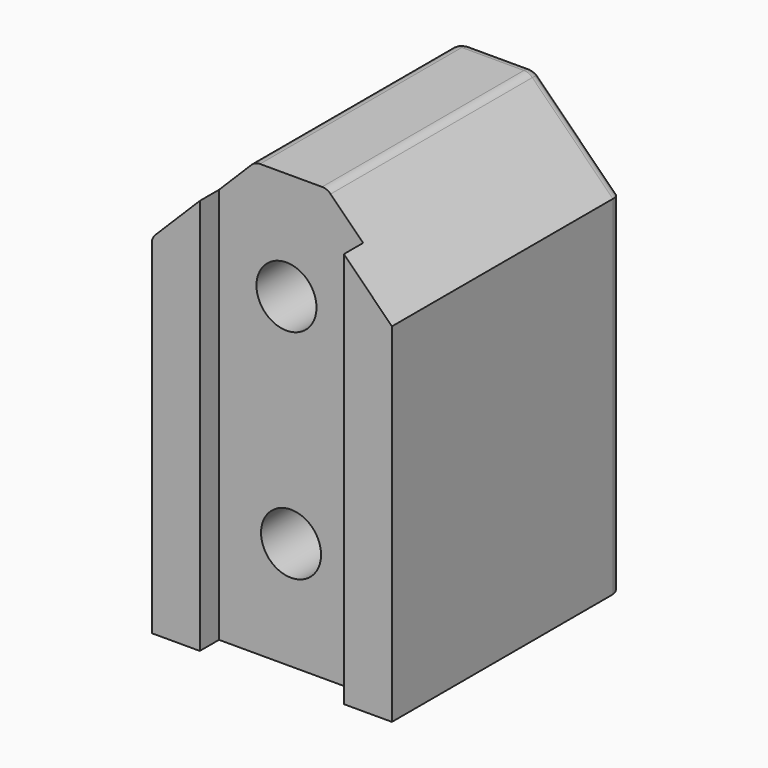
from build123d import *

# Parameters (mm, degrees)
F1_DEPTH    = 12
F2_W        = 6
F2_H        = 22.400515154
F4_DEPTH    = 1
F6_D        = 2.5
F6_DEPTH    = 9.5
F6_TIP      = 0.7510757738
F7_R        = 0.5
F8_T1_DEPTH = 4.7928932188
F8_T3_DEPTH = 6.7426406871
F9_R        = 0.5


# Not quite as in the source:
# - a fillet or chamfer that OpenCascade refuses, or shapes differently, is made with other operations: its cross-section is extruded or revolved along the edge and cut away or added


with BuildPart() as f1:
    # F0 (on Front) → F1 (new body)
    with BuildSketch(Plane.XZ):
        Polygon((0, 14.5), (0, 0), (10, 0), (10, 14.5), (6.5, 18), (3.5, 18), align=None)
    extrude(amount=F1_DEPTH)

    # F2 (on face) → F4 (cut)
    with BuildSketch(Plane.XZ.offset(12)):
        with Locations((5, 11.200257577)):
            Rectangle(F2_W, F2_H)
        Polygon((2, 16.5), (2, 0), (8, 0), (8, 16.5), (6.5, 18), (3.5, 18), align=None)
    extrude(amount=-F4_DEPTH, mode=Mode.SUBTRACT)

    # F6
    with Locations(Plane.XZ.offset(12)):
        with Locations((4.8096684931, 13.5), (5, 4.5)):
            Hole(F6_D / 2, depth=F6_DEPTH)
            with Locations((0, 0, -(F6_DEPTH + F6_TIP / 2))):  # 118° drill point
                Cone(0, F6_D / 2, F6_TIP, mode=Mode.SUBTRACT)

    # F7
    f7_edges = [f1.edges().sort_by_distance(p)[0] for p in [
        (10, 0, 7.25),
        (8.25, 0, 16.25),
        (0, 0, 7.25),
        (5, 0, 0),
    ]]
    fillet(f7_edges, radius=F7_R)

    # F8: fillet of radius 0.5 on 2 edges, made by hand

    # F8_s2 → F8_t1 (cut)
    with BuildSketch(Plane.YZ.offset(2.25)):
        with BuildLine():
            ThreePointArc((0, 17.5), (-0.1464466094, 17.8535533906), (-0.5, 18))
            Line((-0.5, 18), (0, 18))
            Line((0, 18), (0, 17.5))
        make_face()
    extrude(amount=F8_T1_DEPTH, mode=Mode.SUBTRACT)

    # F8_s4 → F8_t3 (cut)
    with BuildSketch(Plane(origin=(11.6338834765, 0, 11.6338834765), x_dir=(0, 1, 0), z_dir=(-0.7071067812, 0, -0.7071067812))):
        with BuildLine():
            ThreePointArc((-0.5, -10.2530483272), (-0.1464466094, -10.1066017178), (0, -9.7530483272))
            Line((0, -9.7530483272), (0, -10.2530483272))
            Line((0, -10.2530483272), (-0.5, -10.2530483272))
        make_face()
    extrude(amount=F8_T3_DEPTH, mode=Mode.SUBTRACT)

    # F9
    f9_edges = [f1.edges().sort_by_distance(p)[0] for p in [
        (3.5, -5.75, 18),
        (0, -6.25, 14.5),
        (6.5, -5.75, 18),
    ]]
    fillet(f9_edges, radius=F9_R)


solid = f1.part
